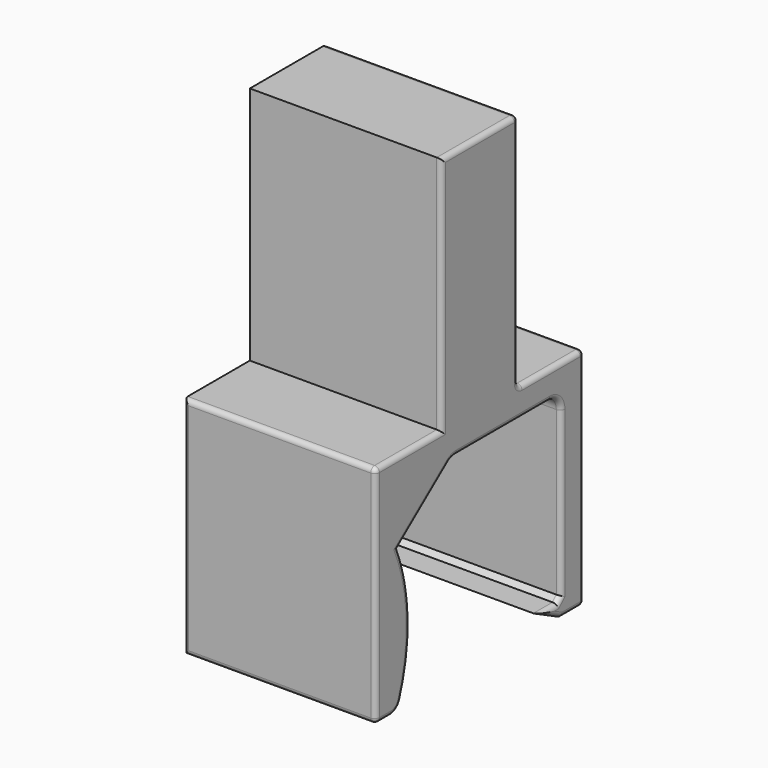
from build123d import *

# Parameters (mm, degrees)
F0_W     = 10
F0_H     = 25
F1_DEPTH = 20
F2_SIZE  = 0.5
F3_R     = 1.5
F4_R     = 0.5


with BuildPart() as f1:
    # F0 (on Right) → F1 (new body)
    with BuildSketch(Plane.YZ):
        Polygon((3, 0), (0, 0), (3, -1.5), align=None)
        Polygon((3, 19), (3, 0), (3, -1.5), (6, -1.5), (6, 22), (-2.6, 22), (-12.6, 22), (-21.2, 22), (-21.2, -1.5), (-18.2, -1.5), (-18.2, 13.5), (-18.2, 19), (-11.2, 19), align=None)
        Polygon((-18.2, 13.5), (-11.2, 19), (-18.2, 19), align=None)
        with BuildLine():
            ThreePointArc((-18.2, -1.5), (-16.7, 6), (-18.2, 13.5))
            Line((-18.2, 13.5), (-18.2, -1.5))
        make_face()
        with Locations((-7.6, 34.5)):
            Rectangle(F0_W, F0_H)
    extrude(amount=F1_DEPTH)

    # F2
    f2_edges = [f1.edges().sort_by_distance(p)[0] for p in [
        (10, 3, 0),
    ]]
    chamfer(f2_edges, length=F2_SIZE)

    # F3
    f3_edges = [f1.edges().sort_by_distance(p)[0] for p in [
        (10, 3, 19),
        (10, -11.2, 19),
        (10, -18.2, -1.5),
    ]]
    fillet(f3_edges, radius=F3_R)

    # F4
    f4_edges = [f1.edges().sort_by_distance(p)[0] for p in [
        (10, -21.2, 22),
        (10, -21.2, -1.5),
        (0, -21.2, 10.25),
        (20, -21.2, 10.25),
        (20, 3, 9),
        (20, 2.56066, 18.56066),
        (20, 2.75, 0.25),
        (20, -4.590603, 19),
        (20, 1.25, 0),
        (20, -11.171503, 18.917606),
        (20, 1.5, -0.75),
        (20, -14.903969, 16.089739),
        (20, 4.5, -1.5),
        (20, -16.707361, 6.535736),
        (20, 6, 10.25),
        (20, -18.363412, -1.224745),
        (20, 1.7, 22),
        (20, -20.214719, -1.5),
        (20, -2.6, 34.5),
        (20, -7.6, 47),
        (20, -16.9, 22),
        (20, -12.6, 34.5),
        (10, 6, -1.5),
        (10, 6, 22),
        (0, 6, 10.25),
        (10, -2.6, 22),
        (10, -2.6, 47),
        (0, -2.6, 34.5),
        (0, 1.7, 22),
    ]]
    fillet(f4_edges, radius=F4_R)


solid = f1.part
